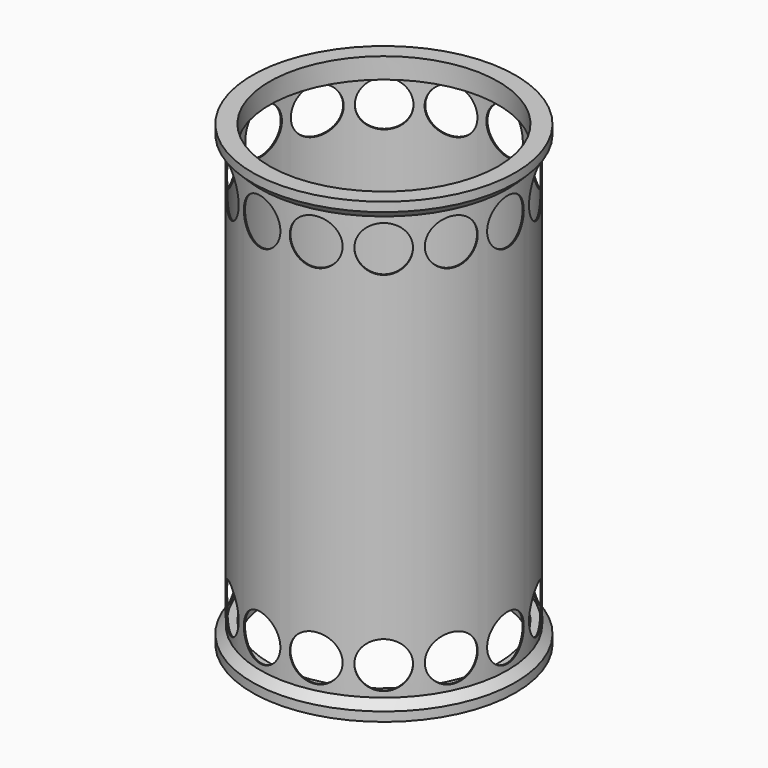
from build123d import *

# Parameters (mm, degrees)
F0_R            = 10.8
F0_R_2          = 10.7
F1_DEPTH        = 20
F1_DEPTH_BACK   = 20
F2_R            = 2
F3_DEPTH        = 25
F3_COPIES_COUNT = 14
F4_R            = 11.5
F4_R_2          = 10
F5_DEPTH        = 1.8
F6_R            = 11.5
F6_R_2          = 10
F7_DEPTH        = 1.8
F8_S5_R         = 10.8
F8_T6_DEPTH     = 18
F8_S11_R        = 10.8
F8_T12_DEPTH    = 18


# Not quite as in the source:
# - a fillet or chamfer that OpenCascade refuses, or shapes differently, is made with other operations: its cross-section is extruded or revolved along the edge and cut away or added
# - a pattern or mirror of a feature is missing from the dataset's text; its kind, count and spacing are read off the source's solid


with BuildPart() as f1:
    # F0 (on Top) → F1 (new body, two sides)
    with BuildSketch(Plane.XY) as f1_sk:
        Circle(F0_R)
        Circle(F0_R_2, mode=Mode.SUBTRACT)
    extrude(amount=F1_DEPTH)
    extrude(f1_sk.sketch, amount=-F1_DEPTH_BACK)

    # F2 (on Right) → F3 (cut)
    with BuildSketch(Plane.YZ):
        with Locations((0, 16)):
            Circle(F2_R)
        with Locations((0, -16)):
            Circle(F2_R)
    f3 = extrude(amount=-F3_DEPTH, mode=Mode.SUBTRACT)

    # F3_copies: F3 ×14 about axis
    f3_copies_axis = Axis((0, 0, 0), (0, 0, 1))
    for i in range(1, F3_COPIES_COUNT):
        add(f3.rotate(f3_copies_axis, i * 360 / F3_COPIES_COUNT), mode=Mode.SUBTRACT)

    # F4 (on face) → F5 (join)
    with BuildSketch(Plane.XY.offset(20)):
        Circle(F4_R)
        Circle(F4_R_2, mode=Mode.SUBTRACT)
    extrude(amount=-F5_DEPTH)

    # F6 (on face) → F7 (join)
    with BuildSketch(Plane(origin=(0, 0, -20), x_dir=(1, 0, 0), z_dir=(0, 0, -1))):
        Circle(F6_R)
        Circle(F6_R_2, mode=Mode.SUBTRACT)
    extrude(amount=-F7_DEPTH)

    # F8: chamfer of 1 on 2 edges, made by hand


with BuildPart() as f8_tool2:
    # F8_s3 → F8_t4 (revolve)
    with BuildSketch(Plane.XZ):
        Polygon((11.5, -19.2), (10.5, -18.2), (11.5, -18.2), align=None)
    revolve(axis=Axis((0, 0, -18.2), (0, 0, -1)))

    # F8_s5 → F8_t6 (cut, symmetric)
    with BuildSketch(Plane.XY.offset(-18.7)):
        Circle(F8_S5_R)
    extrude(amount=F8_T6_DEPTH, both=True, mode=Mode.SUBTRACT)


with BuildPart() as f1_1:
    add(f1.part)

    # F8_t1: cut F8_tool2
    add(f8_tool2.part, mode=Mode.SUBTRACT)


with BuildPart() as f8_tool8:
    # F8_s9 → F8_t10 (revolve)
    with BuildSketch(Plane.XZ):
        Polygon((10.5, 18.2), (11.5, 19.2), (11.5, 18.2), align=None)
    revolve(axis=Axis((0, 0, 18.2), (0, 0, 1)))

    # F8_s11 → F8_t12 (cut, symmetric)
    with BuildSketch(Plane.XY.offset(18.7)):
        Circle(F8_S11_R)
    extrude(amount=F8_T12_DEPTH, both=True, mode=Mode.SUBTRACT)


with BuildPart() as f1_2:
    add(f1_1.part)

    # F8_t7: cut F8_tool8
    add(f8_tool8.part, mode=Mode.SUBTRACT)


solid = f1_2.part
